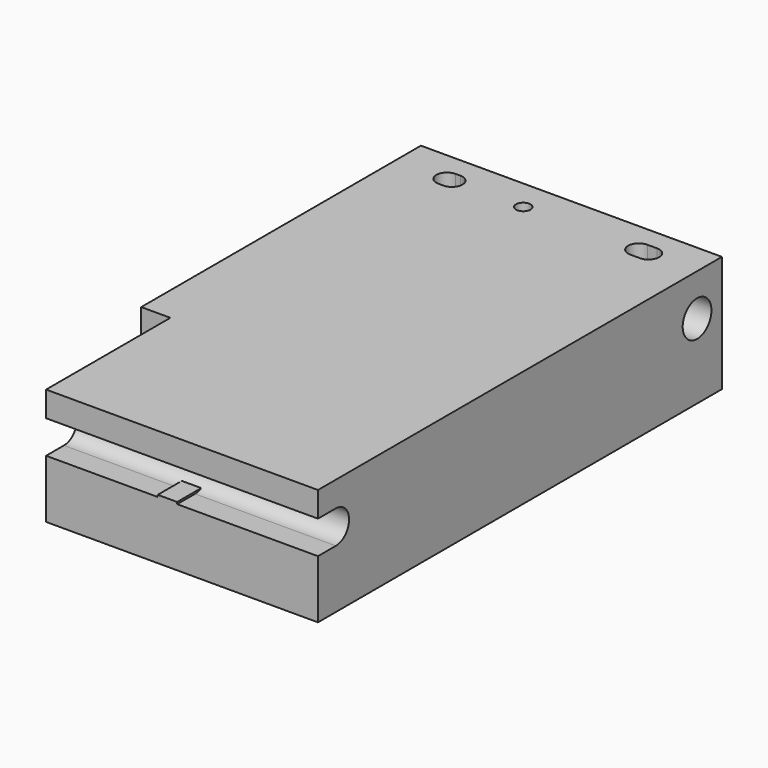
from build123d import *

# Parameters (mm, degrees)
F0_W      = 31
F0_H      = 52
F1_DEPTH  = 12
F2_R      = 1.5
F3_DEPTH  = 25
F4_R      = 0.75
F5_DEPTH  = 2
F6_W      = 2
F6_H      = 0.2
F8_W      = 3
F8_H      = 16
F9_DEPTH  = 12.001
F10_W     = 13
F10_H     = 7
F11_DEPTH = 9.5
F12_R     = 1.85
F12_R_2   = 1.5
F13_DEPTH = 6
F14_R     = 1.85
F15_DEPTH = 6


with BuildPart() as f1:
    # F0 (on Top) → F1 (new body)
    with BuildSketch(Plane.XY):
        Rectangle(F0_W, F0_H)
    extrude(amount=-F1_DEPTH)

    # F2 (on Right) → F3 (cut, symmetric)
    with BuildSketch(Plane.YZ):
        with Locations((22.8, -4.3)):
            Circle(F2_R)
        with BuildLine():
            Line((-28.7, -6), (-23.7, -6))
            ThreePointArc((-23.7, -6), (-22, -4.3), (-23.7, -2.6))
            Line((-23.7, -2.6), (-28.7, -2.6))
            Line((-28.7, -2.6), (-28.7, -6))
        make_face()
    extrude(amount=F3_DEPTH, both=True, mode=Mode.SUBTRACT)

    # F4 (on face) → F5 (cut)
    with BuildSketch(Plane.XY):
        with BuildLine():
            Line((9.5, 21.7), (10.5, 21.7))
            ThreePointArc((10.5, 21.7), (11.6, 22.8), (10.5, 23.9))
            Line((10.5, 23.9), (9.5, 23.9))
            ThreePointArc((9.5, 23.9), (8.4, 22.8), (9.5, 21.7))
        make_face()
        with BuildLine():
            Line((-9.75, 23.9), (-10.25, 23.9))
            ThreePointArc((-10.25, 23.9), (-11.35, 22.8), (-10.25, 21.7))
            Line((-10.25, 21.7), (-9.75, 21.7))
            ThreePointArc((-9.75, 21.7), (-8.65, 22.8), (-9.75, 23.9))
        make_face()
        with Locations((-2.4, 22.8)):
            Circle(F4_R)
    extrude(amount=-F5_DEPTH, mode=Mode.SUBTRACT)

    # F6 (on face) → F7 (join, up to the next surface of F1)
    with BuildSketch(Plane.XZ.offset(26)):
        with Locations((0, -5.9)):
            Rectangle(F6_W, F6_H)
    extrude(until=Until.NEXT, dir=(0, 1, 0))

    # F8 (on face) → F9 (cut, through all)
    with BuildSketch(Plane.XY):
        with Locations((-14, -18)):
            Rectangle(F8_W, F8_H)
    extrude(amount=-F9_DEPTH, mode=Mode.SUBTRACT)

    # F10 (on face) → F11 (cut)
    with BuildSketch(Plane(origin=(0, 0, -12), x_dir=(1, 0, 0), z_dir=(0, 0, -1))):
        with Locations((0, -22.5)):
            Rectangle(F10_W, F10_H)
    extrude(amount=-F11_DEPTH, mode=Mode.SUBTRACT)

    # F12 (on face) → F13 (cut)
    with BuildSketch(Plane(origin=(-15.5, 0, 0), x_dir=(0, -1, 0), z_dir=(-1, 0, 0))):
        with Locations((-22.8, -4.3)):
            Circle(F12_R)
        with Locations((-22.8, -4.3)):
            Circle(F12_R_2, mode=Mode.SUBTRACT)
    extrude(amount=-F13_DEPTH, mode=Mode.SUBTRACT)

    # F14 (on face) → F15 (cut)
    with BuildSketch(Plane.YZ.offset(15.5)):
        with Locations((22.8, -4.3)):
            Circle(F14_R)
    extrude(amount=-F15_DEPTH, mode=Mode.SUBTRACT)


solid = f1.part
